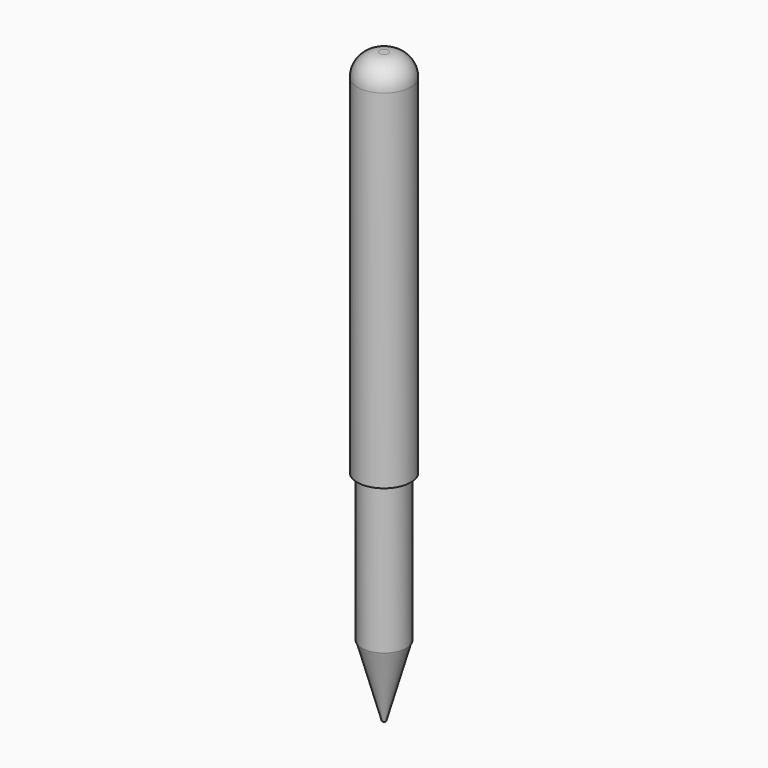
from build123d import *

# Parameters (mm, degrees)
F0_R     = 5
F1_DEPTH = 33
F2_R     = 4.9
F3_DEPTH = 16
F4_SIZE2 = 15.99999
F4_SIZE  = 4.49999
F5_R     = 6
F5_R_2   = 5
F6_DEPTH = 83
F7_R     = 5


# Not quite as in the source:
# - a fillet or chamfer is up to 0.001 mm smaller than in the source, because OpenCascade refuses the exact size


with BuildPart() as f1:
    # F0 (on Top) → F1 (new body)
    with BuildSketch(Plane.XY):
        Circle(F0_R)
    extrude(amount=F1_DEPTH)

    # F2 (on face) → F3 (join)
    with BuildSketch(Plane(origin=(0, 0, 0), x_dir=(1, 0, 0), z_dir=(0, 0, -1))):
        Circle(F2_R)
    extrude(amount=F3_DEPTH)

    # F4 (size 4.5 and 16 in the source; OpenCascade refuses exactly that, so slightly less here)
    f4_edges = [f1.edges().sort_by_distance(p)[0] for p in [
        (-4.9, 0, -16),
    ]]
    f4_side = f1.faces().sort_by_distance((0, 0, -16))[0]
    chamfer(f4_edges, length=F4_SIZE, length2=F4_SIZE2, reference=f4_side)

    # F5 (on face) → F6 (join)
    with BuildSketch(Plane.XY.offset(33)):
        Circle(F5_R)
        Circle(F5_R_2, mode=Mode.SUBTRACT)
        Circle(F5_R_2)
    extrude(amount=F6_DEPTH)

    # F7
    f7_edges = [f1.edges().sort_by_distance(p)[0] for p in [
        (-6, 0, 116),
    ]]
    fillet(f7_edges, radius=F7_R)


solid = f1.part
